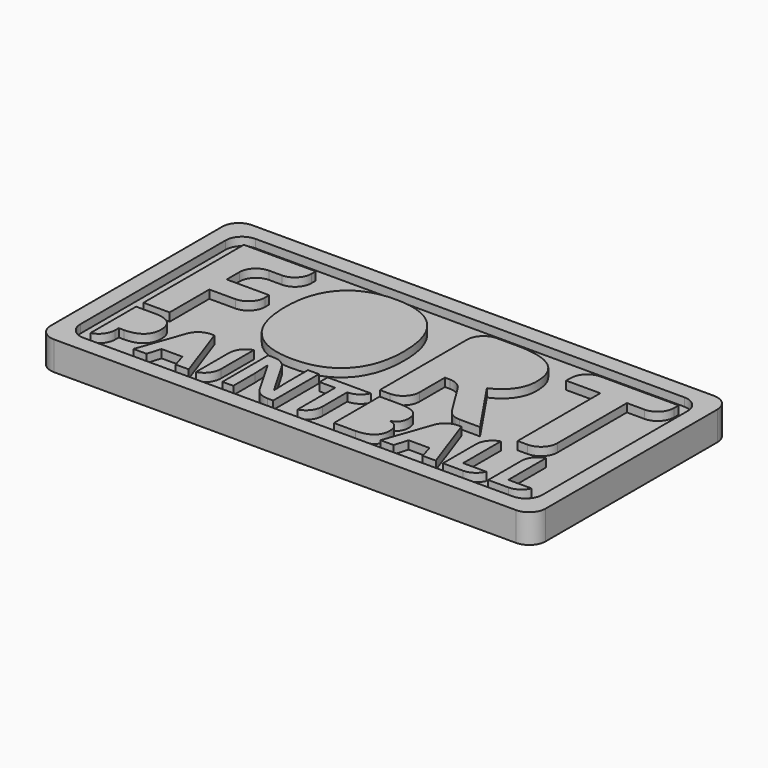
from build123d import *

# Parameters (mm, degrees)
F0_W           = 142.24
F0_H           = 66.04
F0_W_2         = 3.7326379644
F0_H_2         = 17.6000235909
F1_DEPTH       = 6.35
F0_W_3         = 152.4
F0_H_3         = 76.2
F0_TEXT_SIZE   = 54.1061515602
F0_TEXT_SIZE_2 = 24.6531300025
F2_DEPTH       = 8.89
F3_T1_DEPTH    = 2.54
F3_T3_DEPTH    = 15.24
F3_T5_DEPTH    = 9.5947202857
F3_T7_DEPTH    = 11.5370756216
F3_T9_DEPTH    = 14.7851560691
F3_T11_DEPTH   = 14.2406414087
F3_T13_DEPTH   = 9.8858212534
F3_T15_DEPTH   = 9.856957196
F3_T17_DEPTH   = 14.2160872908
F3_T19_DEPTH   = 34.29


# Not quite as in the source:
# - a fillet or chamfer that OpenCascade refuses, or shapes differently, is made with other operations: its cross-section is extruded or revolved along the edge and cut away or added
# - Text() gives the source's letters only with a copy of the font that has no kerning and outlines rounded to 1/6400 em; it was checked with that copy


with BuildPart() as f1:
    # F0 (on Top) → F1 (new body)
    with BuildSketch(Plane.XY):
        Rectangle(F0_W, F0_H)
        with BuildLine():
            add(Edge.make_bspline(
                [(-55.8740079198, -13.8156935938), (-54.2079956188, -15.1947280533), (-54.2079956188, -17.9258326114)],
                knots=[0, 0, 0, 1, 1, 1], degree=2))
            add(Edge.make_bspline(
                [(-54.2079956188, -17.9258326114), (-54.2079956188, -20.7686466648), (-55.9837913893, -22.2728728001)],
                knots=[0, 0, 0, 1, 1, 1], degree=2))
            add(Edge.make_bspline(
                [(-55.9837913893, -22.2728728001), (-57.7595871598, -23.7770989354), (-61.0338309883, -23.7770989354)],
                knots=[0, 0, 0, 1, 1, 1], degree=2))
            Line((-61.0338309883, -23.7770989354), (-62.6324323869, -23.7770989354))
            Line((-62.6324323869, -23.7770989354), (-62.6324323869, -30.0366827251))
            Line((-62.6324323869, -30.0366827251), (-66.3650703513, -30.0366827251))
            Line((-66.3650703513, -30.0366827251), (-66.3650703513, -12.4366591343))
            Line((-66.3650703513, -12.4366591343), (-60.7449271211, -12.4366591343))
            add(Edge.make_bspline(
                [(-60.7449271211, -12.4366591343), (-57.5400202207, -12.4366591343), (-55.8740079198, -13.8156935938)],
                knots=[0, 0, 0, 1, 1, 1], degree=2))
        make_face(mode=Mode.SUBTRACT)
        Polygon((-36.087945067, -30.0366827251), (-40.1094868986, -30.0366827251), (-41.384515966, -25.8456506247), (-47.8020338697, -25.8456506247), (-49.0770629371, -30.0366827251), (-53.0986047687, -30.0366827251), (-46.8852455978, -12.3634701546), (-42.3244165473, -12.3634701546), align=None, mode=Mode.SUBTRACT)
        with Locations((-32.0066964361, -21.2366709297)):
            Rectangle(F0_W_2, F0_H_2, mode=Mode.SUBTRACT)
        with BuildLine():
            Line((-10.0981531721, -12.4366591343), (-10.0981531721, -30.0366827251))
            Line((-10.0981531721, -30.0366827251), (-14.8400286461, -30.0366827251))
            Line((-14.8400286461, -30.0366827251), (-22.4979071531, -16.7239925238))
            Line((-22.4979071531, -16.7239925238), (-22.6057645968, -16.7239925238))
            add(Edge.make_bspline(
                [(-22.6057645968, -16.7239925238), (-22.3746415031, -20.2486197038), (-22.3746415031, -21.7547718649)],
                knots=[0, 0, 0, 1, 1, 1], degree=2))
            Line((-22.3746415031, -21.7547718649), (-22.3746415031, -30.0366827251))
            Line((-22.3746415031, -30.0366827251), (-25.7105181565, -30.0366827251))
            Line((-25.7105181565, -30.0366827251), (-25.7105181565, -12.4366591343))
            Line((-25.7105181565, -12.4366591343), (-21.0033111467, -12.4366591343))
            Line((-21.0033111467, -12.4366591343), (-13.3608408459, -25.6183795825))
            Line((-13.3608408459, -25.6183795825), (-13.2760957115, -25.6183795825))
            add(Edge.make_bspline(
                [(-13.2760957115, -25.6183795825), (-13.457142135, -22.18620164), (-13.457142135, -20.7686466648)],
                knots=[0, 0, 0, 1, 1, 1], degree=2))
            Line((-13.457142135, -20.7686466648), (-13.457142135, -12.4366591343))
            Line((-13.457142135, -12.4366591343), (-10.0981531721, -12.4366591343))
        make_face(mode=Mode.SUBTRACT)
        Polygon((1.1228730306, -15.541412694), (1.1228730306, -30.0366827251), (-2.6097649339, -30.0366827251), (-2.6097649339, -15.541412694), (-7.3901609234, -15.541412694), (-7.3901609234, -12.4366591343), (5.8994169686, -12.4366591343), (5.8994169686, -15.541412694), align=None, mode=Mode.SUBTRACT)
        with BuildLine():
            Line((8.6074092173, -30.0366827251), (8.6074092173, -12.4366591343))
            Line((8.6074092173, -12.4366591343), (14.0850265397, -12.4366591343))
            add(Edge.make_bspline(
                [(14.0850265397, -12.4366591343), (17.8292206589, -12.4366591343), (19.520271295, -13.5017513914)],
                knots=[0, 0, 0, 1, 1, 1], degree=2))
            add(Edge.make_bspline(
                [(19.520271295, -13.5017513914), (21.2113219311, -14.5668436486), (21.2113219311, -16.889630741)],
                knots=[0, 0, 0, 1, 1, 1], degree=2))
            add(Edge.make_bspline(
                [(21.2113219311, -16.889630741), (21.2113219311, -18.4689718818), (20.471728031, -19.480135417)],
                knots=[0, 0, 0, 1, 1, 1], degree=2))
            add(Edge.make_bspline(
                [(20.471728031, -19.480135417), (19.7321341309, -20.4912989523), (18.5033296824, -20.6954576851)],
                knots=[0, 0, 0, 1, 1, 1], degree=2))
            Line((18.5033296824, -20.6954576851), (18.5033296824, -20.8148712836))
            add(Edge.make_bspline(
                [(18.5033296824, -20.8148712836), (20.1751200607, -21.1885202852), (20.9166399865, -22.2112399751)],
                knots=[0, 0, 0, 1, 1, 1], degree=2))
            add(Edge.make_bspline(
                [(20.9166399865, -22.2112399751), (21.6581599124, -23.2339596651), (21.6581599124, -24.9327144043)],
                knots=[0, 0, 0, 1, 1, 1], degree=2))
            add(Edge.make_bspline(
                [(21.6581599124, -24.9327144043), (21.6581599124, -27.3402466311), (19.9170326059, -28.6884646781)],
                knots=[0, 0, 0, 1, 1, 1], degree=2))
            add(Edge.make_bspline(
                [(19.9170326059, -28.6884646781), (18.1759052995, -30.0366827251), (15.1905653383, -30.0366827251)],
                knots=[0, 0, 0, 1, 1, 1], degree=2))
            Line((15.1905653383, -30.0366827251), (8.6074092173, -30.0366827251))
        make_face(mode=Mode.SUBTRACT)
        Polygon((39.9669609908, -30.0366827251), (35.9454191592, -30.0366827251), (34.6703900918, -25.8456506247), (28.2528721881, -25.8456506247), (26.9778431207, -30.0366827251), (22.9563012891, -30.0366827251), (29.16966046, -12.3634701546), (33.7304895105, -12.3634701546), align=None, mode=Mode.SUBTRACT)
        Polygon((53.05238015, -30.0366827251), (42.1818906395, -30.0366827251), (42.1818906395, -12.4366591343), (45.9145286039, -12.4366591343), (45.9145286039, -26.9550414748), (53.05238015, -26.9550414748), align=None, mode=Mode.SUBTRACT)
        Polygon((66.9813986014, -30.0366827251), (56.1109090909, -30.0366827251), (56.1109090909, -12.4366591343), (59.8435470554, -12.4366591343), (59.8435470554, -26.9550414748), (66.9813986014, -26.9550414748), align=None, mode=Mode.SUBTRACT)
        Polygon((-58.202156315, 5.5216505201), (-58.202156315, -9.7464291233), (-66.2589004458, -9.7464291233), (-66.2589004458, 28.8802906389), (-44.117648737, 28.8802906389), (-44.117648737, 22.167746211), (-58.202156315, 22.167746211), (-58.202156315, 12.2088326895), (-45.098322734, 12.2088326895), (-45.098322734, 5.5216505201), align=None, mode=Mode.SUBTRACT)
        with BuildLine():
            add(Edge.make_bspline(
                [(-6.2179803863, 24.361581575), (-1.5006002972, 19.2341783061), (-1.5006002972, 9.621882318)],
                knots=[0, 0, 0, 1, 1, 1], degree=2))
            add(Edge.make_bspline(
                [(-1.5006002972, 9.621882318), (-1.5006002972, 0.0264945022), (-6.2560237741, -5.1262710253)],
                knots=[0, 0, 0, 1, 1, 1], degree=2))
            add(Edge.make_bspline(
                [(-6.2560237741, -5.1262710253), (-11.0114472511, -10.2790365527), (-19.8882377415, -10.2790365527)],
                knots=[0, 0, 0, 1, 1, 1], degree=2))
            add(Edge.make_bspline(
                [(-19.8882377415, -10.2790365527), (-28.7650282318, -10.2790365527), (-33.5204517088, -5.1262710253)],
                knots=[0, 0, 0, 1, 1, 1], degree=2))
            add(Edge.make_bspline(
                [(-33.5204517088, -5.1262710253), (-38.2758751857, 0.0264945022), (-38.2758751857, 9.6726068351)],
                knots=[0, 0, 0, 1, 1, 1], degree=2))
            add(Edge.make_bspline(
                [(-38.2758751857, 9.6726068351), (-38.2758751857, 19.3187191679), (-33.5077705795, 24.4038520059)],
                knots=[0, 0, 0, 1, 1, 1], degree=2))
            add(Edge.make_bspline(
                [(-33.5077705795, 24.4038520059), (-28.7396659733, 29.488984844), (-19.8375132244, 29.488984844)],
                knots=[0, 0, 0, 1, 1, 1], degree=2))
            add(Edge.make_bspline(
                [(-19.8375132244, 29.488984844), (-10.9353604755, 29.488984844), (-6.2179803863, 24.361581575)],
                knots=[0, 0, 0, 1, 1, 1], degree=2))
        make_face(mode=Mode.SUBTRACT)
        with BuildLine():
            Line((19.0512832095, 5.0735839525), (14.6974288262, 5.0735839525))
            Line((14.6974288262, 5.0735839525), (14.6974288262, -9.7464291233))
            Line((14.6974288262, -9.7464291233), (6.5054193165, -9.7464291233))
            Line((6.5054193165, -9.7464291233), (6.5054193165, 28.8802906389))
            Line((6.5054193165, 28.8802906389), (17.7578080238, 28.8802906389))
            add(Edge.make_bspline(
                [(17.7578080238, 28.8802906389), (25.6370163447, 28.8802906389), (29.4117658247, 26.0143554235)],
                knots=[0, 0, 0, 1, 1, 1], degree=2))
            add(Edge.make_bspline(
                [(29.4117658247, 26.0143554235), (33.1865153046, 23.148420208), (33.1865153046, 17.3066466568)],
                knots=[0, 0, 0, 1, 1, 1], degree=2))
            add(Edge.make_bspline(
                [(33.1865153046, 17.3066466568), (33.1865153046, 13.8996499257), (31.3139352155, 11.2450668648)],
                knots=[0, 0, 0, 1, 1, 1], degree=2))
            add(Edge.make_bspline(
                [(31.3139352155, 11.2450668648), (29.4413551263, 8.5904838039), (26.0005420505, 7.0856564636)],
                knots=[0, 0, 0, 1, 1, 1], degree=2))
            add(Edge.make_bspline(
                [(26.0005420505, 7.0856564636), (34.7251589896, -5.9420903418), (37.3628338782, -9.7464291233)],
                knots=[0, 0, 0, 1, 1, 1], degree=2))
            Line((37.3628338782, -9.7464291233), (28.2746912333, -9.7464291233))
            Line((28.2746912333, -9.7464291233), (19.0512832095, 5.0735839525))
        make_face(mode=Mode.SUBTRACT)
        Polygon((57.12848737, 22.0662971768), (57.12848737, -9.7464291233), (48.9364778603, -9.7464291233), (48.9364778603, 22.0662971768), (38.4449569094, 22.0662971768), (38.4449569094, 28.8802906389), (67.6115542348, 28.8802906389), (67.6115542348, 22.0662971768), align=None, mode=Mode.SUBTRACT)
    extrude(amount=F1_DEPTH)

    # F0 (on Top) → F2 (join)
    with BuildSketch(Plane.XY):
        Rectangle(F0_W_3, F0_H_3)
        Rectangle(F0_W, F0_H, mode=Mode.SUBTRACT)
        with Locations((-71.12, -9.7464291233)):
            Text('FORT', F0_TEXT_SIZE, font='Open Sans', font_style=FontStyle.BOLD, text_align=(TextAlign.LEFT, TextAlign.BOTTOM))
        with BuildLine():
            add(Edge.make_bspline(
                [(-27.2052493314, 19.3778977712), (-29.6865236256, 16.0892582467), (-29.6865236256, 9.621882318)],
                knots=[0, 0, 0, 1, 1, 1], degree=2))
            add(Edge.make_bspline(
                [(-29.6865236256, 9.621882318), (-29.6865236256, 3.1460523031), (-27.2306115899, -0.1299060921)],
                knots=[0, 0, 0, 1, 1, 1], degree=2))
            add(Edge.make_bspline(
                [(-27.2306115899, -0.1299060921), (-24.7746995542, -3.4058644874), (-19.8882377415, -3.4058644874)],
                knots=[0, 0, 0, 1, 1, 1], degree=2))
            add(Edge.make_bspline(
                [(-19.8882377415, -3.4058644874), (-10.0899518574, -3.4058644874), (-10.0899518574, 9.621882318)],
                knots=[0, 0, 0, 1, 1, 1], degree=2))
            add(Edge.make_bspline(
                [(-10.0899518574, 9.621882318), (-10.0899518574, 22.6665372957), (-19.8375132244, 22.6665372957)],
                knots=[0, 0, 0, 1, 1, 1], degree=2))
            add(Edge.make_bspline(
                [(-19.8375132244, 22.6665372957), (-24.7239750371, 22.6665372957), (-27.2052493314, 19.3778977712)],
                knots=[0, 0, 0, 1, 1, 1], degree=2))
        make_face()
        with BuildLine():
            Line((14.6974288262, 22.167746211), (14.6974288262, 11.7354038633))
            Line((14.6974288262, 11.7354038633), (17.3351037147, 11.7354038633))
            add(Edge.make_bspline(
                [(17.3351037147, 11.7354038633), (21.2239833581, 11.7354038633), (23.0712011887, 13.028879049)],
                knots=[0, 0, 0, 1, 1, 1], degree=2))
            add(Edge.make_bspline(
                [(23.0712011887, 13.028879049), (24.9184190193, 14.3223542348), (24.9184190193, 17.0952945022)],
                knots=[0, 0, 0, 1, 1, 1], degree=2))
            add(Edge.make_bspline(
                [(24.9184190193, 17.0952945022), (24.9184190193, 19.8428725111), (23.0289307578, 21.0053093611)],
                knots=[0, 0, 0, 1, 1, 1], degree=2))
            add(Edge.make_bspline(
                [(23.0289307578, 21.0053093611), (21.1394424963, 22.167746211), (17.1829301634, 22.167746211)],
                knots=[0, 0, 0, 1, 1, 1], degree=2))
            Line((17.1829301634, 22.167746211), (14.6974288262, 22.167746211))
        make_face()
        with Locations((-68.58, -30.0366827251)):
            Text('PAINTBALL', F0_TEXT_SIZE_2, font='Open Sans', font_style=FontStyle.BOLD, text_align=(TextAlign.LEFT, TextAlign.BOTTOM))
        with BuildLine():
            Line((14.6512781195, -22.3672480634), (12.3400471817, -22.3672480634))
            Line((12.3400471817, -22.3672480634), (12.3400471817, -26.9550414748))
            Line((12.3400471817, -26.9550414748), (14.7706917179, -26.9550414748))
            add(Edge.make_bspline(
                [(14.7706917179, -26.9550414748), (16.3115123431, -26.9550414748), (17.0453281658, -26.3656775857)],
                knots=[0, 0, 0, 1, 1, 1], degree=2))
            add(Edge.make_bspline(
                [(17.0453281658, -26.3656775857), (17.7791439885, -25.7763136966), (17.7791439885, -24.5590654027)],
                knots=[0, 0, 0, 1, 1, 1], degree=2))
            add(Edge.make_bspline(
                [(17.7791439885, -24.5590654027), (17.7791439885, -22.3672480634), (14.6512781195, -22.3672480634)],
                knots=[0, 0, 0, 1, 1, 1], degree=2))
        make_face()
        with BuildLine():
            Line((-62.6324323869, -15.4951880752), (-62.6324323869, -20.7185699945))
            Line((-62.6324323869, -20.7185699945), (-61.4036279383, -20.7185699945))
            add(Edge.make_bspline(
                [(-61.4036279383, -20.7185699945), (-59.6856129413, -20.7185699945), (-58.8304574943, -20.0386828937)],
                knots=[0, 0, 0, 1, 1, 1], degree=2))
            add(Edge.make_bspline(
                [(-58.8304574943, -20.0386828937), (-57.9753020474, -19.3587957928), (-57.9753020474, -18.0606544161)],
                knots=[0, 0, 0, 1, 1, 1], degree=2))
            add(Edge.make_bspline(
                [(-57.9753020474, -18.0606544161), (-57.9753020474, -16.7471048332), (-58.691783638, -16.1211464542)],
                knots=[0, 0, 0, 1, 1, 1], degree=2))
            add(Edge.make_bspline(
                [(-58.691783638, -16.1211464542), (-59.4082652287, -15.4951880752), (-60.9375296992, -15.4951880752)],
                knots=[0, 0, 0, 1, 1, 1], degree=2))
            Line((-60.9375296992, -15.4951880752), (-62.6324323869, -15.4951880752))
        make_face()
        with BuildLine():
            Line((12.3400471817, -15.4951880752), (12.3400471817, -19.4088724631))
            Line((12.3400471817, -19.4088724631), (14.5049001601, -19.4088724631))
            add(Edge.make_bspline(
                [(14.5049001601, -19.4088724631), (16.0226084759, -19.4088724631), (16.7024955767, -18.9389221724)],
                knots=[0, 0, 0, 1, 1, 1], degree=2))
            add(Edge.make_bspline(
                [(16.7024955767, -18.9389221724), (17.3823826776, -18.4689718818), (17.3823826776, -17.3865453926)],
                knots=[0, 0, 0, 1, 1, 1], degree=2))
            add(Edge.make_bspline(
                [(17.3823826776, -17.3865453926), (17.3823826776, -16.3734558316), (16.6427887775, -15.9343219534)],
                knots=[0, 0, 0, 1, 1, 1], degree=2))
            add(Edge.make_bspline(
                [(16.6427887775, -15.9343219534), (15.9031948774, -15.4951880752), (14.3007414272, -15.4951880752)],
                knots=[0, 0, 0, 1, 1, 1], degree=2))
            Line((14.3007414272, -15.4951880752), (12.3400471817, -15.4951880752))
        make_face()
        with BuildLine():
            Line((29.1927727694, -22.7177847556), (33.7767141292, -22.7177847556))
            add(Edge.make_bspline(
                [(33.7767141292, -22.7177847556), (32.0086224619, -17.0244525457), (31.7852034712, -16.2771545425)],
                knots=[0, 0, 0, 1, 1, 1], degree=2))
            add(Edge.make_bspline(
                [(31.7852034712, -16.2771545425), (31.5617844806, -15.5298565393), (31.4654831915, -15.0984267642)],
                knots=[0, 0, 0, 1, 1, 1], degree=2))
            add(Edge.make_bspline(
                [(31.4654831915, -15.0984267642), (31.0687218805, -16.6392473894), (29.1927727694, -22.7177847556)],
                knots=[0, 0, 0, 1, 1, 1], degree=2))
        make_face()
        with BuildLine():
            Line((-46.8621332884, -22.7177847556), (-42.2781919286, -22.7177847556))
            add(Edge.make_bspline(
                [(-42.2781919286, -22.7177847556), (-44.0462835959, -17.0244525457), (-44.2697025866, -16.2771545425)],
                knots=[0, 0, 0, 1, 1, 1], degree=2))
            add(Edge.make_bspline(
                [(-44.2697025866, -16.2771545425), (-44.4931215772, -15.5298565393), (-44.5894228663, -15.0984267642)],
                knots=[0, 0, 0, 1, 1, 1], degree=2))
            add(Edge.make_bspline(
                [(-44.5894228663, -15.0984267642), (-44.9861841773, -16.6392473894), (-46.8621332884, -22.7177847556)],
                knots=[0, 0, 0, 1, 1, 1], degree=2))
        make_face()
    extrude(amount=F2_DEPTH)

    # F3: fillet of radius 5.08 on 31 edges, made by hand

    # F3_s2 → F3_t1 (join)
    with BuildSketch(Plane.XY.offset(6.35)):
        with BuildLine():
            ThreePointArc((-58.202156315, 17.087746211), (-56.7142587634, 20.6798486594), (-53.122156315, 22.167746211))
            Line((-53.122156315, 22.167746211), (-58.202156315, 22.167746211))
            Line((-58.202156315, 22.167746211), (-58.202156315, 17.087746211))
        make_face()
        with BuildLine():
            ThreePointArc((20.5423328527, 2.6777910793), (18.6962379961, 4.434426902), (16.2293950952, 5.0735839525))
            Line((16.2293950952, 5.0735839525), (19.0512832095, 5.0735839525))
            Line((19.0512832095, 5.0735839525), (20.5423328527, 2.6777910793))
        make_face()
        with BuildLine():
            ThreePointArc((-71.12, -27.94), (-69.6321024484, -31.5321024484), (-66.04, -33.02))
            Line((-66.04, -33.02), (-71.12, -33.02))
            Line((-71.12, -33.02), (-71.12, -27.94))
        make_face()
        with BuildLine():
            ThreePointArc((71.12, 27.94), (69.6321024484, 31.5321024484), (66.04, 33.02))
            Line((66.04, 33.02), (71.12, 33.02))
            Line((71.12, 33.02), (71.12, 27.94))
        make_face()
        with BuildLine():
            ThreePointArc((-71.12, 27.94), (-69.6321024484, 31.5321024484), (-66.04, 33.02))
            Line((-66.04, 33.02), (-71.12, 33.02))
            Line((-71.12, 33.02), (-71.12, 27.94))
        make_face()
        with BuildLine():
            ThreePointArc((66.04, -33.02), (69.6321024484, -31.5321024484), (71.12, -27.94))
            Line((71.12, -27.94), (71.12, -33.02))
            Line((71.12, -33.02), (66.04, -33.02))
        make_face()
    extrude(amount=F3_T1_DEPTH)

    # F3_s4 → F3_t3 (cut)
    with BuildSketch(Plane.XY.offset(6.35)):
        with BuildLine():
            ThreePointArc((57.12848737, -4.6664291233), (55.6405898184, -8.2585315718), (52.04848737, -9.7464291233))
            Line((52.04848737, -9.7464291233), (57.12848737, -9.7464291233))
            Line((57.12848737, -9.7464291233), (57.12848737, -4.6664291233))
        make_face()
        with BuildLine():
            ThreePointArc((43.5249569094, 28.8802906389), (39.9328544609, 27.3923930874), (38.4449569094, 23.8002906389))
            Line((38.4449569094, 23.8002906389), (38.4449569094, 28.8802906389))
            Line((38.4449569094, 28.8802906389), (43.5249569094, 28.8802906389))
        make_face()
        with BuildLine():
            ThreePointArc((62.5315542348, 22.0662971768), (66.1236566832, 23.5541947284), (67.6115542348, 27.1462971768))
            Line((67.6115542348, 27.1462971768), (67.6115542348, 22.0662971768))
            Line((67.6115542348, 22.0662971768), (62.5315542348, 22.0662971768))
        make_face()
        with BuildLine():
            ThreePointArc((11.5854193165, 28.8802906389), (7.9933168681, 27.3923930874), (6.5054193165, 23.8002906389))
            Line((6.5054193165, 23.8002906389), (6.5054193165, 28.8802906389))
            Line((6.5054193165, 28.8802906389), (11.5854193165, 28.8802906389))
        make_face()
        with BuildLine():
            ThreePointArc((9.6174288262, -9.7464291233), (13.2095312746, -8.2585315718), (14.6974288262, -4.6664291233))
            Line((14.6974288262, -4.6664291233), (14.6974288262, -9.7464291233))
            Line((14.6974288262, -9.7464291233), (9.6174288262, -9.7464291233))
        make_face()
        with BuildLine():
            ThreePointArc((-49.197648737, 22.167746211), (-45.6055462886, 23.6556437626), (-44.117648737, 27.247746211))
            Line((-44.117648737, 27.247746211), (-44.117648737, 22.167746211))
            Line((-44.117648737, 22.167746211), (-49.197648737, 22.167746211))
        make_face()
        with BuildLine():
            ThreePointArc((-50.178322734, 5.5216505201), (-46.5862202856, 7.0095480716), (-45.098322734, 10.6016505201))
            Line((-45.098322734, 10.6016505201), (-45.098322734, 5.5216505201))
            Line((-45.098322734, 5.5216505201), (-50.178322734, 5.5216505201))
        make_face()
    extrude(amount=F3_T3_DEPTH, mode=Mode.SUBTRACT)

    # F3_s6 → F3_t5 (cut)
    with BuildSketch(Plane.XY.offset(6.35)):
        with BuildLine():
            ThreePointArc((26.7836415901, -7.3506362502), (28.6297364467, -9.1072720728), (31.0965793476, -9.7464291233))
            Line((31.0965793476, -9.7464291233), (28.2746912333, -9.7464291233))
            Line((28.2746912333, -9.7464291233), (26.7836415901, -7.3506362502))
        make_face()
    extrude(amount=F3_T5_DEPTH, mode=Mode.SUBTRACT)

    # F3_s8 → F3_t7 (cut)
    with BuildSketch(Plane.XY.offset(6.35)):
        with BuildLine():
            ThreePointArc((-43.2864153491, -12.3634701546), (-46.2230134391, -13.298257053), (-48.0788660881, -15.7585915491))
            Line((-48.0788660881, -15.7585915491), (-46.8852455978, -12.3634701546))
            Line((-46.8852455978, -12.3634701546), (-43.2864153491, -12.3634701546))
        make_face()
        with BuildLine():
            ThreePointArc((32.7684907087, -12.3634701546), (29.8318926187, -13.298257053), (27.9760399697, -15.7585915491))
            Line((27.9760399697, -15.7585915491), (29.16966046, -12.3634701546))
            Line((29.16966046, -12.3634701546), (32.7684907087, -12.3634701546))
        make_face()
    extrude(amount=F3_T7_DEPTH, mode=Mode.SUBTRACT)

    # F3_s10 → F3_t9 (cut)
    with BuildSketch(Plane.XY.offset(6.35)):
        with BuildLine():
            ThreePointArc((-33.8730154183, -17.3347215619), (-32.8334980096, -14.2556144787), (-30.1403774539, -12.4366591343))
            Line((-30.1403774539, -12.4366591343), (-33.8730154183, -12.4366591343))
            Line((-33.8730154183, -12.4366591343), (-33.8730154183, -17.3347215619))
        make_face()
        with BuildLine():
            ThreePointArc((-33.8730154183, -30.0366827251), (-31.1798948626, -28.2177273807), (-30.1403774539, -25.1386202975))
            Line((-30.1403774539, -25.1386202975), (-30.1403774539, -30.0366827251))
            Line((-30.1403774539, -30.0366827251), (-33.8730154183, -30.0366827251))
        make_face()
        with BuildLine():
            ThreePointArc((1.1228730306, -25.1386202975), (0.0833556218, -28.2177273807), (-2.6097649339, -30.0366827251))
            Line((-2.6097649339, -30.0366827251), (1.1228730306, -30.0366827251))
            Line((1.1228730306, -30.0366827251), (1.1228730306, -25.1386202975))
        make_face()
        with BuildLine():
            ThreePointArc((42.1818906395, -17.3347215619), (43.2214080482, -14.2556144787), (45.9145286039, -12.4366591343))
            Line((45.9145286039, -12.4366591343), (42.1818906395, -12.4366591343))
            Line((42.1818906395, -12.4366591343), (42.1818906395, -17.3347215619))
        make_face()
        with BuildLine():
            ThreePointArc((56.1109090909, -17.3347215619), (57.1504264996, -14.2556144787), (59.8435470554, -12.4366591343))
            Line((59.8435470554, -12.4366591343), (56.1109090909, -12.4366591343))
            Line((56.1109090909, -12.4366591343), (56.1109090909, -17.3347215619))
        make_face()
        with BuildLine():
            ThreePointArc((-62.6324323869, -25.1386202975), (-63.6719497956, -28.2177273807), (-66.3650703513, -30.0366827251))
            Line((-66.3650703513, -30.0366827251), (-62.6324323869, -30.0366827251))
            Line((-62.6324323869, -30.0366827251), (-62.6324323869, -25.1386202975))
        make_face()
    extrude(amount=F3_T9_DEPTH, mode=Mode.SUBTRACT)

    # F3_s12 → F3_t11 (cut)
    with BuildSketch(Plane.XY.offset(6.35)):
        with BuildLine():
            ThreePointArc((1.2191604051, -15.541412694), (4.0273758601, -14.6946532917), (5.8994169686, -12.4366591343))
            Line((5.8994169686, -12.4366591343), (5.8994169686, -15.541412694))
            Line((5.8994169686, -15.541412694), (1.2191604051, -15.541412694))
        make_face()
    extrude(amount=F3_T11_DEPTH, mode=Mode.SUBTRACT)

    # F3_s14 → F3_t13 (cut)
    with BuildSketch(Plane.XY.offset(6.35)):
        with BuildLine():
            ThreePointArc((-11.9017001447, -30.0366827251), (-14.4451980783, -29.3540703885), (-16.305143623, -27.4896820408))
            Line((-16.305143623, -27.4896820408), (-14.8400286461, -30.0366827251))
            Line((-14.8400286461, -30.0366827251), (-11.9017001447, -30.0366827251))
        make_face()
    extrude(amount=F3_T13_DEPTH, mode=Mode.SUBTRACT)

    # F3_s16 → F3_t15 (cut)
    with BuildSketch(Plane.XY.offset(6.35)):
        with BuildLine():
            ThreePointArc((-19.535312038, -14.9686616292), (-21.3940959302, -13.1149420076), (-23.9300940251, -12.4366591343))
            Line((-23.9300940251, -12.4366591343), (-21.0033111467, -12.4366591343))
            Line((-21.0033111467, -12.4366591343), (-19.535312038, -14.9686616292))
        make_face()
    extrude(amount=F3_T15_DEPTH, mode=Mode.SUBTRACT)

    # F3_s18 → F3_t17 (cut)
    with BuildSketch(Plane.XY.offset(6.35)):
        with BuildLine():
            ThreePointArc((48.3819452337, -30.0366827251), (51.1796887487, -29.1968514982), (53.05238015, -26.9550414748))
            Line((53.05238015, -26.9550414748), (53.05238015, -30.0366827251))
            Line((53.05238015, -30.0366827251), (48.3819452337, -30.0366827251))
        make_face()
        with BuildLine():
            ThreePointArc((62.3109636851, -30.0366827251), (65.1087072001, -29.1968514982), (66.9813986014, -26.9550414748))
            Line((66.9813986014, -26.9550414748), (66.9813986014, -30.0366827251))
            Line((66.9813986014, -30.0366827251), (62.3109636851, -30.0366827251))
        make_face()
    extrude(amount=F3_T17_DEPTH, mode=Mode.SUBTRACT)

    # F3_s20 → F3_t19 (cut)
    with BuildSketch(Plane.XY.offset(-12.7)):
        with BuildLine():
            ThreePointArc((-71.12, -38.1), (-74.7121024484, -36.6121024484), (-76.2, -33.02))
            Line((-76.2, -33.02), (-76.2, -38.1))
            Line((-76.2, -38.1), (-71.12, -38.1))
        make_face()
        with BuildLine():
            ThreePointArc((-71.12, 38.1), (-74.7121024484, 36.6121024484), (-76.2, 33.02))
            Line((-76.2, 33.02), (-76.2, 38.1))
            Line((-76.2, 38.1), (-71.12, 38.1))
        make_face()
        with BuildLine():
            ThreePointArc((71.12, -38.1), (74.7121024484, -36.6121024484), (76.2, -33.02))
            Line((76.2, -33.02), (76.2, -38.1))
            Line((76.2, -38.1), (71.12, -38.1))
        make_face()
        with BuildLine():
            ThreePointArc((76.2, 33.02), (74.7121024484, 36.6121024484), (71.12, 38.1))
            Line((71.12, 38.1), (76.2, 38.1))
            Line((76.2, 38.1), (76.2, 33.02))
        make_face()
    extrude(amount=F3_T19_DEPTH, mode=Mode.SUBTRACT)


solid = f1.part
